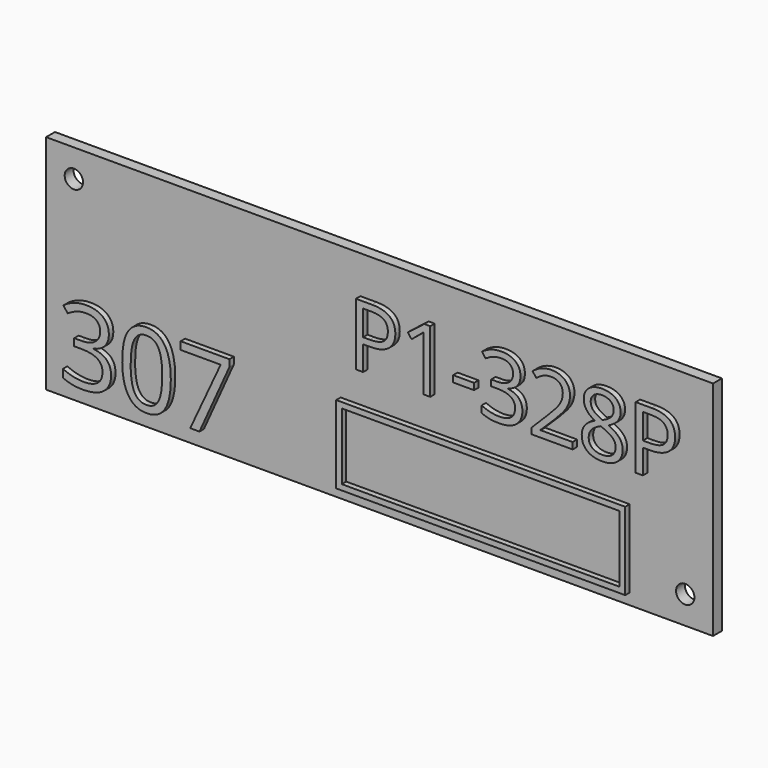
from build123d import *

# Parameters (mm, degrees)
F0_W         = 120
F0_H         = 40
F1_DEPTH     = 2
F3_D         = 3.3
F4_TEXT_SIZE = 15.681149951
F5_DEPTH     = 1
F6_TEXT_SIZE = 18.5054667028
F7_DEPTH     = 1
F8_W         = 52
F8_H         = 14
F8_W_2       = 49.99999962
F8_H_2       = 11.99999962
F9_DEPTH     = 1


# Not quite as in the source:
# - Text() gives the source's letters only with a copy of the font that has no kerning and outlines rounded to 1/6400 em; it was checked with that copy


with BuildPart() as f1:
    # F0 (on Front) → F1 (new body)
    with BuildSketch(Plane.XZ):
        Rectangle(F0_W, F0_H)
    extrude(amount=F1_DEPTH)

    # F3 (through all)
    with Locations(Plane.XZ.offset(2)):
        with Locations((-55, 15), (55, -15)):
            Hole(F3_D / 2)

    # F4 (on face) → F5 (join)
    with BuildSketch(Plane.XZ.offset(2)):
        with Locations((-5, 2)):
            Text('P1-328P', F4_TEXT_SIZE, font='Open Sans', text_align=(TextAlign.LEFT, TextAlign.BOTTOM))
    extrude(amount=F5_DEPTH)

    # F6 (on face) → F7 (join)
    with BuildSketch(Plane.XZ.offset(2)):
        with Locations((-57, -17)):
            Text('307', F6_TEXT_SIZE, font='Open Sans', text_align=(TextAlign.LEFT, TextAlign.BOTTOM))
    extrude(amount=F7_DEPTH)

    # F8 (on face) → F9 (join)
    with BuildSketch(Plane.XZ.offset(2)):
        with Locations((19, -11)):
            Rectangle(F8_W, F8_H)
        with Locations((19, -11)):
            Rectangle(F8_W_2, F8_H_2, mode=Mode.SUBTRACT)
    extrude(amount=F9_DEPTH)


solid = f1.part
